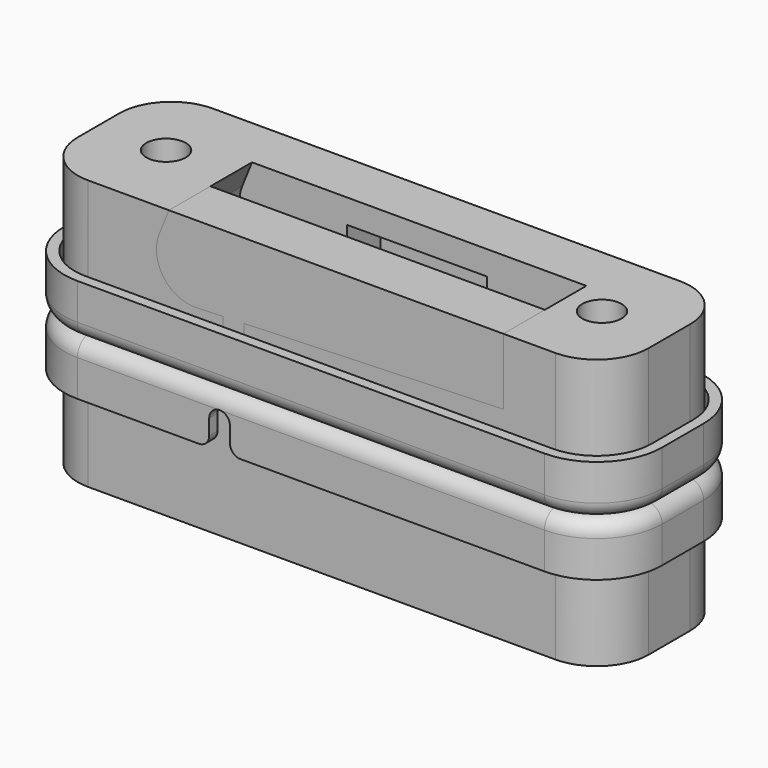
from build123d import *

# Parameters (mm, degrees)
F1_DEPTH       = 13
F2_D           = 3.8
F2_CSINK_D     = 10
F2_CSINK_ANGLE = 90
F3_D           = 3.8
F3_CSINK_D     = 10
F3_CSINK_ANGLE = 90
F5_DEPTH       = 10
F7_DEPTH       = 13.001
F9_SIZE        = 1
F10_R          = 2.0203490491
F11_DEPTH      = 2
F13_DEPTH      = 4
F15_DEPTH      = 3
F8_W           = 2
F8_H           = 15
F16_DEPTH      = 2
F20_DEPTH      = 5
F21_T          = -1
F22_W          = 2
F22_H          = 3.5
F23_DEPTH      = 1
F24_R          = 0.99999
F25_R          = 1.49999


# Not quite as in the source:
# - a fillet or chamfer is up to 0.001 mm smaller than in the source, because OpenCascade refuses the exact size


with BuildPart() as f1:
    # F0 (on Top) → F1 (new body)
    with BuildSketch(Plane.XY):
        with BuildLine():
            Line((22.5, 7.5), (-22.5, 7.5))
            ThreePointArc((-22.5, 7.5), (-26.0355339059, 6.0355339059), (-27.5, 2.5))
            Line((-27.5, 2.5), (-27.5, -2.5))
            ThreePointArc((-27.5, -2.5), (-26.0355339059, -6.0355339059), (-22.5, -7.5))
            Line((-22.5, -7.5), (22.5, -7.5))
            ThreePointArc((22.5, -7.5), (26.0355339059, -6.0355339059), (27.5, -2.5))
            Line((27.5, -2.5), (27.5, 2.5))
            ThreePointArc((27.5, 2.5), (26.0355339059, 6.0355339059), (22.5, 7.5))
        make_face()
    extrude(amount=-F1_DEPTH)

    # F2 (through all)
    with Locations(Plane.XY):
        with Locations((-21, 0)):
            CounterSinkHole(F2_D / 2, F2_CSINK_D / 2, counter_sink_angle=F2_CSINK_ANGLE)

    # F3 (through all)
    with Locations(Plane.XY):
        with Locations((21, 0)):
            CounterSinkHole(F3_D / 2, F3_CSINK_D / 2, counter_sink_angle=F3_CSINK_ANGLE)

    # F4 (on face) → F5 (cut)
    with BuildSketch(Plane(origin=(0, 7.5, 0), x_dir=(-1, 0, 0), z_dir=(0, 1, 0))):
        with BuildLine():
            Line((-17.5, -6.6), (-17.5, -13))
            Line((-17.5, -13), (12.1, -13))
            Line((12.1, -13), (12.35, -13))
            Line((12.35, -13), (14.7179837091, -13))
            Line((14.7179837091, -13), (15.6549660938, -10.693182542))
            ThreePointArc((15.6549660938, -10.693182542), (15.2607581132, -7.1810857313), (12.1, -5.6))
            Line((12.1, -5.6), (2.2234824646, -5.933666133))
            Line((2.2234824646, -5.933666133), (1.2314146634, -5.967181937))
            Line((1.2314146634, -5.967181937), (-17.5, -6.6))
        make_face()
    extrude(amount=-F5_DEPTH, mode=Mode.SUBTRACT)

    # F6 (on face) → F7 (cut, through all)
    with BuildSketch(Plane.XY):
        with BuildLine():
            Line((-7.5, 4.4860103474), (-7.5, 7.5))
            Line((-7.5, 7.5), (-9.5, 7.5))
            Line((-9.5, 7.5), (-9.5, 4.4860103474))
            ThreePointArc((-9.5, 4.4860103474), (-8.5, 0.2764359465), (-7.5, 4.4860103474))
        make_face()
    extrude(amount=-F7_DEPTH, mode=Mode.SUBTRACT)

    # F9
    f9_edges = [f1.edges().sort_by_distance(p)[0] for p in [
        (-16, 7.5, 0),
    ]]
    chamfer(f9_edges, length=F9_SIZE)

    # F10 (on face) → F11 (cut)
    with BuildSketch(Plane(origin=(-0.2027680241, 0, -6.0019335127), x_dir=(0.999429816, 0, -0.0337645208), z_dir=(-0.0337645208, 0, -0.999429816))):
        with Locations((-8.3019656238, -2.5)):
            Circle(F10_R)
    extrude(amount=-F11_DEPTH, mode=Mode.SUBTRACT)

    # F12 (on face) → F13 (cut)
    with BuildSketch(Plane(origin=(0, -2.5, 0), x_dir=(-1, 0, 0), z_dir=(0, 1, 0))):
        Polygon((5.5504581337, -5.8212683063), (-7.9315317385, -6.2767409371), (-7.9315317385, -10.6757969008), (5.5504581337, -10.6757969008), align=None)
    extrude(amount=-F13_DEPTH, mode=Mode.SUBTRACT)

    # F14 (on face) → F15 (cut)
    with BuildSketch(Plane(origin=(-0.2027680241, 0, -6.0019335127), x_dir=(0.999429816, 0, -0.0337645208), z_dir=(-0.0337645208, 0, -0.999429816))):
        with BuildLine():
            Line((14.9289605508, -0.2764359465), (-8.3019656238, -0.2764359465))
            Line((-8.3019656238, -0.2764359465), (-8.3019656238, -4.2764359465))
            Line((-8.3019656238, -4.2764359465), (14.9289605508, -4.2764359465))
            ThreePointArc((14.9289605508, -4.2764359465), (15.6360673319, -3.9835427277), (15.9289605508, -3.2764359465))
            Line((15.9289605508, -3.2764359465), (15.9289605508, -1.2764359465))
            ThreePointArc((15.9289605508, -1.2764359465), (15.6360673319, -0.5693291653), (14.9289605508, -0.2764359465))
        make_face()
    extrude(amount=-F15_DEPTH, mode=Mode.SUBTRACT)

    # F8 (on face) → F16 (cut)
    with BuildSketch(Plane.XY):
        with Locations((-8.5, 0)):
            Rectangle(F8_W, F8_H)
    extrude(amount=-F16_DEPTH, mode=Mode.SUBTRACT)


with BuildPart() as f17_1:
    # F17: instance of F1
    add(f1.part.mirror(Plane.XY))


with BuildPart() as f18_1:
    # F18: instance of F17_1
    add(f17_1.part.mirror(Plane.XZ))


with BuildPart() as f20:
    # F19 (on face) → F20 (new body)
    with BuildSketch(Plane.XY):
        with BuildLine():
            ThreePointArc((-22.5, 8.8), (-26.9547727215, 6.9547727215), (-28.8, 2.5))
            Line((-28.8, 2.5), (-28.8, -2.5))
            ThreePointArc((-28.8, -2.5), (-26.9547727215, -6.9547727215), (-22.5, -8.8))
            Line((-22.5, -8.8), (22.5, -8.8))
            ThreePointArc((22.5, -8.8), (26.9547727215, -6.9547727215), (28.8, -2.5))
            Line((28.8, -2.5), (28.8, 2.5))
            ThreePointArc((28.8, 2.5), (26.9547727215, 6.9547727215), (22.5, 8.8))
            Line((22.5, 8.8), (-22.5, 8.8))
        make_face()
    extrude(amount=-F20_DEPTH)

    # F21
    f21_openings = [f20.faces().sort_by_distance(p)[0] for p in [
        (0, 0, -5),
    ]]
    offset(amount=F21_T, openings=f21_openings)

    # F22 (on face) → F23 (cut, through all)
    with BuildSketch(Plane.XZ.offset(8.8)):
        with Locations((-8.8, -3.25)):
            Rectangle(F22_W, F22_H)
    extrude(amount=-F23_DEPTH, mode=Mode.SUBTRACT)

    # F24 (radius 1 in the source; OpenCascade refuses exactly that, so slightly less here)
    f24_edges = [f20.edges().sort_by_distance(p)[0] for p in [
        (-9.8, -8.3, -5),
        (-7.8, -8.3, -5),
        (-9.8, -8.3, -1.5),
        (-7.8, -8.3, -1.5),
    ]]
    fillet(f24_edges, radius=F24_R)

    # F25 (radius 1.5 in the source; OpenCascade refuses exactly that, so slightly less here)
    f25_edges = [f20.edges().sort_by_distance(p)[0] for p in [
        (0, -8.8, 0),
    ]]
    fillet(f25_edges, radius=F25_R)


with BuildPart() as f26_1:
    # F26: instance of F20
    add(f20.part.mirror(Plane.XY))


with BuildPart() as f27_1:
    # F27: instance of F26_1
    add(f26_1.part.mirror(Plane.XZ))


solid = Compound([f1.part, f17_1.part, f18_1.part, f20.part, f26_1.part, f27_1.part])
